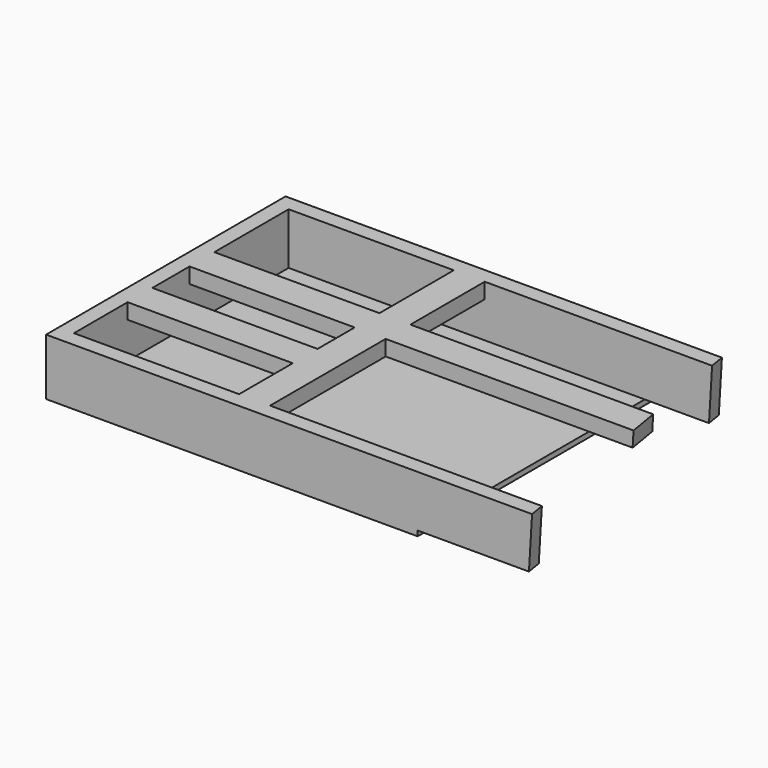
from build123d import *

# Parameters (mm, degrees)
F0_W          = 457.2
F0_H          = 368.3
F1_DEPTH      = 6.35
F2_W          = 19.05
F2_H          = 330.2
F2_W_2        = 177.8
F2_H_2        = 19.05
F3_DEPTH      = 63.5
F4_W          = 203.2
F4_H          = 38.1
F4_W_2        = 374.65
F5_DEPTH      = 19.05
F8_DEPTH      = 125.9670187868
F8_DEPTH_BACK = 65.6385295619


# Not quite as in the source:
# - a feature names something its author has since deleted; it is built from what else it names


with BuildPart() as f1:
    # F0 (on Top) → F1 (new body)
    with BuildSketch(Plane.XY):
        with Locations((228.6, 184.15)):
            Rectangle(F0_W, F0_H)
    extrude(amount=F1_DEPTH)

    # F2 (on face) → F3 (join)
    with BuildSketch(Plane.XY.offset(6.35)):
        with Locations((9.525, 184.15)):
            Rectangle(F2_W, F2_H)
        Polygon((0, 368.3), (0, 349.25), (19.05, 349.25), (457.2, 349.25), (457.2, 368.3), align=None)
        Polygon((0, 19.05), (0, 0), (457.2, 0), (457.2, 19.05), (19.05, 19.05), align=None)
        with Locations((546.1, 9.525)):
            Rectangle(F2_W_2, F2_H_2)
        with Locations((546.1, 358.775)):
            Rectangle(F2_W_2, F2_H_2)
    extrude(amount=F3_DEPTH)

    # F4 (on face) → F5 (join)
    with BuildSketch(Plane.XY.offset(69.85)):
        with Locations((120.65, 120.65)):
            Rectangle(F4_W, F4_H)
        Polygon((222.25, 101.6), (222.25, 19.05), (260.35, 19.05), (260.35, 196.85), (260.35, 234.95), (260.35, 349.25), (222.25, 349.25), (222.25, 234.95), (222.25, 196.85), (222.25, 139.7), align=None)
        with Locations((120.65, 215.9)):
            Rectangle(F4_W, F4_H)
        with Locations((447.675, 215.9)):
            Rectangle(F4_W_2, F4_H)
    extrude(amount=-F5_DEPTH)

    # F7 (on face) → F8 (cut, two sides)
    with BuildSketch(Plane(origin=(0, 22.4493572683, 61.6791021759), x_dir=(1, 0, 0), z_dir=(0, -0.3420201433, -0.9396926208))) as f8_sk:
        Polygon((643.6106, 282.7225558054), (513.744137013, -453.7867547107), (643.6106, -453.7867547107), align=None)
    extrude(amount=-F8_DEPTH, mode=Mode.SUBTRACT)
    extrude(f8_sk.sketch, amount=F8_DEPTH_BACK, mode=Mode.SUBTRACT)


solid = f1.part
